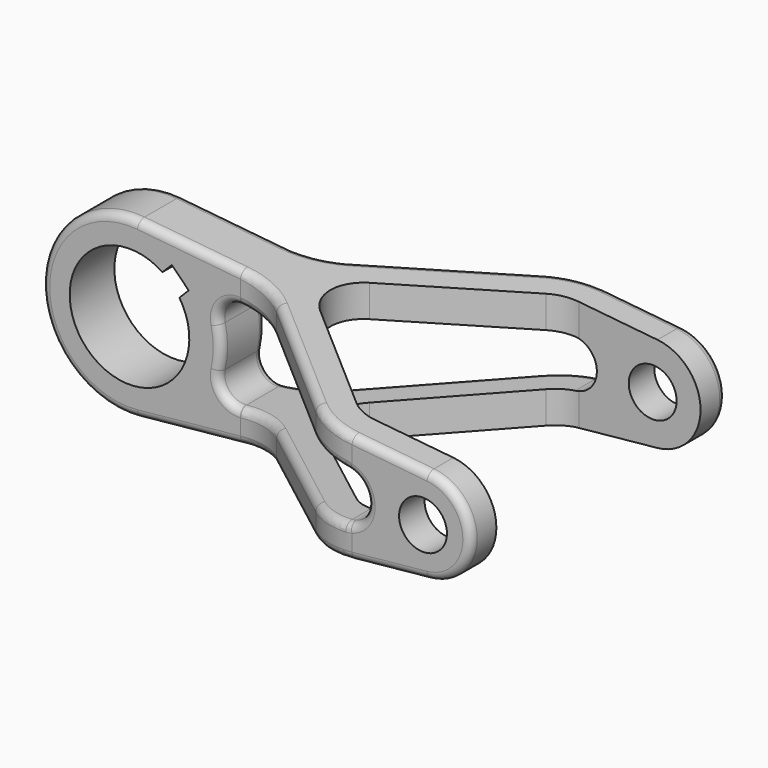
from build123d import *

# Parameters (mm, degrees)
F0_R          = 6
F1_DEPTH      = 40
F3_DEPTH      = 22.001
F3_DEPTH_BACK = 22.001
F4_R          = 10
F5_R          = 20
F6_R          = 2


# Not quite as in the source:
# - a pattern or mirror of a feature is missing from the dataset's text; its kind, count and spacing are read off the source's solid


with BuildPart() as f1:
    # F0 (on Front) → F1 (new body, symmetric)
    with BuildSketch(Plane.XZ):
        with BuildLine():
            Line((101.2, 11.9398492453), (2.2, 21.8897236163))
            ThreePointArc((2.2, 21.8897236163), (-22, 0), (2.2, -21.8897236163))
            Line((2.2, -21.8897236163), (101.2, -11.9398492453))
            ThreePointArc((101.2, -11.9398492453), (112, 0), (101.2, 11.9398492453))
        make_face()
        with BuildLine():
            ThreePointArc((12.513625189, 8.2709845019), (-10.6066017178, -10.6066017178), (8.2709845019, 12.513625189))
            Line((8.2709845019, 12.513625189), (10.6066017178, 14.8492424049))
            Line((10.6066017178, 14.8492424049), (14.8492424049, 10.6066017178))
            Line((14.8492424049, 10.6066017178), (12.513625189, 8.2709845019))
        make_face(mode=Mode.SUBTRACT)
        with BuildLine():
            ThreePointArc((27.7812433369, -11.2784094028), (23.5286399945, -9.6077070992), (22.409592741, -5.1778521785))
            ThreePointArc((22.409592741, -5.1778521785), (23, 0), (22.409592741, 5.1778521785))
            ThreePointArc((22.409592741, 5.1778521785), (23.5286399945, 9.6077070992), (27.7812433369, 11.2784094028))
            Line((27.7812433369, 11.2784094028), (80.6, 5.9699246226))
            ThreePointArc((80.6, 5.9699246226), (86, 0), (80.6, -5.9699246226))
            Line((80.6, -5.9699246226), (27.7812433369, -11.2784094028))
        make_face(mode=Mode.SUBTRACT)
        with Locations((100, 0)):
            Circle(F0_R, mode=Mode.SUBTRACT)
    extrude(amount=F1_DEPTH, both=True)

    # F2 (on Top) → F3 (cut, two sides)
    with BuildSketch(Plane.XY) as f3_sk:
        Polygon((-22, 40), (-22, 7), (35, 7), (75, 40), align=None)
        Polygon((112, 0), (112, 32), (77.8740772485, 32), (39.0861984606, 0), align=None)
    f3 = extrude(amount=-F3_DEPTH, mode=Mode.SUBTRACT) + extrude(f3_sk.sketch, amount=F3_DEPTH_BACK, mode=Mode.SUBTRACT)

    # F3_copies: F3 across plane
    add(f3.mirror(Plane(origin=(0, 0, 0), x_dir=(0, 0, -1), z_dir=(0, -1, 0))), mode=Mode.SUBTRACT)

    # F4
    f4_edges = [f1.edges().sort_by_distance(p)[0] for p in [
        (77.874077, 32, 10.264041),
        (77.874077, 32, -10.264041),
        (77.874077, -32, 10.264041),
        (39.086198, 0, 14.16237),
        (39.086198, 0, -14.16237),
        (77.874077, -32, -10.264041),
    ]]
    fillet(f4_edges, radius=F4_R)

    # F5
    f5_edges = [f1.edges().sort_by_distance(p)[0] for p in [
        (75, 40, 10.552897),
        (75, 40, -10.552897),
        (35, 7, -14.573048),
        (35, 7, 14.573048),
        (75, -40, -10.552897),
        (75, -40, 10.552897),
        (35, -7, -14.573048),
        (35, -7, 14.573048),
    ]]
    fillet(f5_edges, radius=F5_R)

    # F6
    f6_edges = [f1.edges().sort_by_distance(p)[0] for p in [
        (-22, 7, 0),
        (34.573431, 8.176584, 10.595769),
        (91.692597, -40, -12.895379),
        (75.423141, -38.822185, -14.530521),
        (55, -23.5, -16.583124),
        (34.576859, -8.177815, -18.635727),
        (15.007403, -7, -20.602531),
        (15.007403, 7, -20.602531),
        (34.576859, 8.177815, -18.635727),
        (55, 23.5, -16.583124),
        (75.423141, 38.822185, -14.530521),
        (91.692597, 40, -12.895379),
        (86, -40, 0),
        (91.692597, -40, 12.895379),
        (112, -40, 0),
        (81.415687, -39.985191, -5.830594),
        (74.681954, -38.539186, -6.564711),
        (55, -23.5, -8.542821),
        (34.576859, -8.177815, -10.595424),
        (15.007403, -7, 20.602531),
        (-22, -7, 0),
        (27.798025, -7, 11.276723),
        (23.52864, -7, 9.607707),
        (23, -7, 0),
        (27.798025, -7, -11.276723),
        (23.52864, -7, -9.607707),
        (15.007403, 7, 20.602531),
        (27.798025, 7, 11.276723),
        (23.52864, 7, 9.607707),
        (23, 7, 0),
        (27.798025, 7, -11.276723),
        (23.52864, 7, -9.607707),
        (34.576859, 8.177815, -10.595424),
        (55, 23.5, -8.542821),
        (74.681954, 38.539186, -6.564711),
        (81.415687, 39.985191, -5.830594),
        (112, 40, 0),
        (86, 40, 0),
        (91.692597, 40, 12.895379),
        (81.415699, -39.985192, 5.830591),
        (74.681954, -38.539186, 6.564711),
        (75.423141, -38.822185, 14.530521),
        (75.423141, 38.822185, 14.530521),
        (55, 23.5, 16.583124),
        (34.576859, 8.177815, 18.635727),
        (34.576859, -8.177815, 18.635727),
        (55, -23.5, 16.583124),
        (34.576859, -8.177815, 10.595424),
        (55, -23.5, 8.542821),
        (74.681954, 38.539186, 6.564711),
        (55, 23.5, 8.542821),
        (81.415699, 39.985192, 5.830591),
    ]]
    fillet(f6_edges, radius=F6_R)


solid = f1.part
